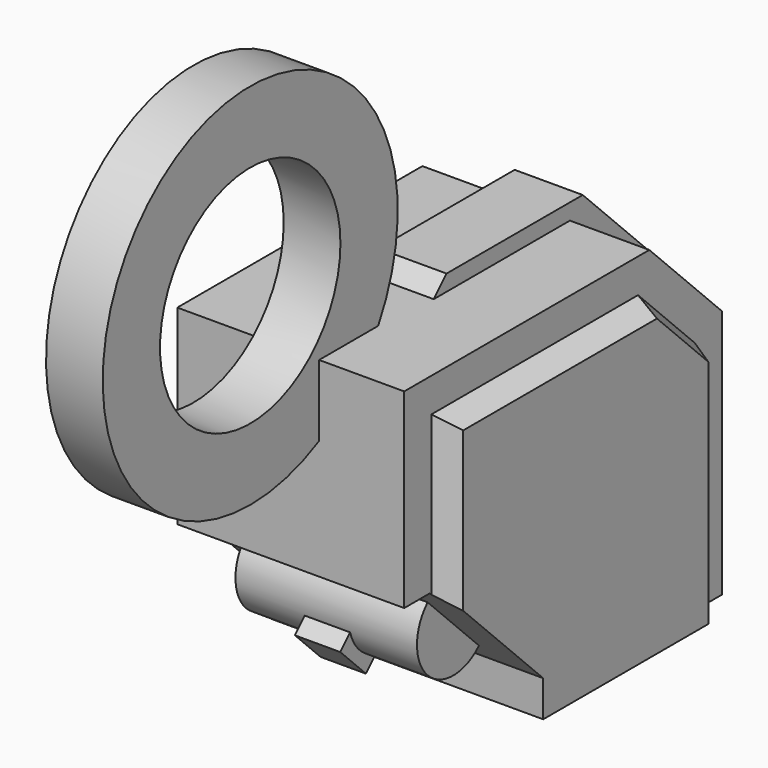
from build123d import *

# Parameters (mm, degrees)
F2_DEPTH       = 20
F3_DEPTH       = 22
F3_DEPTH_BACK  = 2
F1_W           = 29
F1_H           = 3
F7_DEPTH       = 22
F7_DEPTH_BACK  = 2
F5_W           = 6
F5_H           = 11.313708499
F4_W           = 6
F4_H           = 15
F6_W           = 6
F6_H           = 15
F8_DEPTH       = 2
F10_DEPTH      = 25
F12_DEPTH      = 5
F15_DEPTH      = 0.5
F16_R          = 16.2487088964
F16_R_2        = 9.9373882072
F17_DEPTH      = 2.5
F17_DEPTH_BACK = 2.5
F18_T4_DEPTH   = 31.116674808
F18_T9_DEPTH   = 19.1877426199
F18_T14_DEPTH  = 33.116674808
F18_T19_DEPTH  = 24.3595810189
F18_T24_DEPTH  = 24.3595810189
F18_T29_DEPTH  = 33.116674808
F18_T34_DEPTH  = 19.1877426199
F18_T39_DEPTH  = 31.116674808


# Not quite as in the source:
# - a fillet or chamfer that OpenCascade refuses, or shapes differently, is made with other operations: its cross-section is extruded or revolved along the edge and cut away or added
# - two fillets or chamfers of one size are made in one step


with BuildPart() as f2:
    # F1 (on Right) → F2 (new body)
    with BuildSketch(Plane.YZ):
        Polygon((-35, 30), (-35, 0), (-32, 0), (-32, 3), (-32, 27), (-9.2426406871, 27), (-3, 20.7573593129), (-3, 3), (-3, 0), (0, 0), (0, 22), (-8, 30), align=None)
    extrude(amount=F2_DEPTH)

    # F1 (on Right) → F3 (join, two sides)
    with BuildSketch(Plane.YZ) as f3_sk:
        Polygon((-32, 27), (-32, 3), (-3, 3), (-3, 20.7573593129), (-9.2426406871, 27), align=None)
    extrude(amount=F3_DEPTH)
    extrude(f3_sk.sketch, amount=-F3_DEPTH_BACK)

    # F1 (on Right) → F7 (join, two sides)
    with BuildSketch(Plane.YZ) as f7_sk:
        with Locations((-17.5, 1.5)):
            Rectangle(F1_W, F1_H)
    extrude(amount=F7_DEPTH)
    extrude(f7_sk.sketch, amount=-F7_DEPTH_BACK)

    # F5 (on face) + F4 (on face) + F6 (on face) → F8 (join)
    with BuildSketch(Plane(origin=(0, 11, 11), x_dir=(-1, 0, 0), z_dir=(0, 0.7071067812, 0.7071067812))):
        with Locations((-10, 21.2132034356)):
            Rectangle(F5_W, F5_H)
    with BuildSketch(Plane(origin=(0, 0, 0), x_dir=(-1, 0, 0), z_dir=(0, 1, 0))):
        with Locations((-10, 14.5)):
            Rectangle(F4_W, F4_H)
    with BuildSketch(Plane.XY.offset(30)):
        with Locations((10, -15.5)):
            Rectangle(F6_W, F6_H)
    extrude(amount=F8_DEPTH, dir=(0, 0.7071067812, 0.7071067812))

    # F9 (on face) → F10 (cut)
    with BuildSketch(Plane(origin=(-2, 0, 0), x_dir=(0, -1, 0), z_dir=(-1, 0, 0))):
        Polygon((22.18895033, -6.8113151938), (42.18895033, -6.8113151938), (42.18895033, 13.1886848062), (32.18895033, 13.1886848062), (32, 12.9997344762), (32, 0), (22.18895033, 0), align=None)
        Polygon((22.18895033, 3.1886848062), (22.18895033, 0), (32, 0), (32, 12.9997344762), align=None)
    extrude(amount=-F10_DEPTH, mode=Mode.SUBTRACT)

    # F11 (on face) → F12 (join)
    with BuildSketch(Plane(origin=(0, -9.5001327619, -9.5001327619), x_dir=(1, 0, 0), z_dir=(0, -0.7071067812, -0.7071067812))):
        Polygon((8, 26.8821576475), (8, 24.8821576475), (8, 22.8821576475), (12, 22.8821576475), (12, 24.8821576475), (12, 26.8821576475), align=None)
    extrude(amount=F12_DEPTH)

    # F11 (on face) → F13 (revolve)
    with BuildSketch(Plane(origin=(0, -9.5001327619, -9.5001327619), x_dir=(1, 0, 0), z_dir=(0, -0.7071067812, -0.7071067812))):
        Polygon((2, 28.8821576475), (2, 24.8821576475), (8, 24.8821576475), (8, 26.8821576475), (12, 26.8821576475), (12, 24.8821576475), (18, 24.8821576475), (18, 28.8821576475), align=None)
    revolve(axis=Axis((5, -27.094475165, 8.0942096412), (1, 0, 0)))

    # F14 (on face) → F15 (join)
    with BuildSketch(Plane(origin=(0, 1.4142135624, 0), x_dir=(-1, 0, 0), z_dir=(0, 1, 0))):
        with BuildLine():
            Line((-12, 21.4142135624), (-12, 10.4142135624))
            ThreePointArc((-12, 10.4142135624), (-11.7071067812, 9.7071067812), (-11, 9.4142135624))
            Line((-11, 9.4142135624), (-9, 9.4142135624))
            ThreePointArc((-9, 9.4142135624), (-8.2928932188, 9.7071067812), (-8, 10.4142135624))
            Line((-8, 10.4142135624), (-8, 21.4142135624))
            ThreePointArc((-8, 21.4142135624), (-8.2928932188, 22.1213203436), (-9, 22.4142135624))
            Line((-9, 22.4142135624), (-11, 22.4142135624))
            ThreePointArc((-11, 22.4142135624), (-11.7071067812, 22.1213203436), (-12, 21.4142135624))
        make_face()
    extrude(amount=F15_DEPTH)

    # F16 (on offset) → F17 (join, two sides)
    with BuildSketch(Plane.YZ.offset(10)) as f17_sk:
        with Locations((-42.5896607339, 38.0838625133)):
            Circle(F16_R)
        with Locations((-42.5896607339, 38.0838625133)):
            Circle(F16_R_2, mode=Mode.SUBTRACT)
    extrude(amount=F17_DEPTH)
    extrude(f17_sk.sketch, amount=-F17_DEPTH_BACK)

    # F18: chamfer of 2 x 1 on 8 edges, made by hand


with BuildPart() as f18_tool2:
    # F18_s3 → F18_t4 (new body)
    with BuildSketch(Plane.XY.offset(-5.1796577476)):
        Polygon((0, -3), (-2, -4), (-2, -3), align=None)
    extrude(amount=F18_T4_DEPTH)

    split(bisect_by=Plane.YZ, keep=Keep.BOTTOM)


with BuildPart() as f2_1:
    add(f2.part)

    # F18_t1: cut F18_tool2
    add(f18_tool2.part, mode=Mode.SUBTRACT)


with BuildPart() as f18_tool7:
    # F18_s8 → F18_t9 (new body)
    with BuildSketch(Plane(origin=(0, -8.2161085389, 8.2161085389), x_dir=(1, 0, 0), z_dir=(0, -0.7071067812, 0.7071067812))):
        Polygon((0, 12.5563491861), (-2, 11.5563491861), (-2, 12.5563491861), align=None)
    extrude(amount=F18_T9_DEPTH)

    split(bisect_by=Plane.YZ, keep=Keep.BOTTOM)


with BuildPart() as f2_2:
    add(f2_1.part)

    # F18_t6: cut F18_tool7
    add(f18_tool7.part, mode=Mode.SUBTRACT)


with BuildPart() as f18_tool12:
    # F18_s13 → F18_t14 (new body)
    with BuildSketch(Plane.XZ.offset(4.0629829395)):
        Polygon((0, 27), (-2, 26), (-2, 27), align=None)
    extrude(amount=F18_T14_DEPTH)

    split(bisect_by=Plane.YZ, keep=Keep.BOTTOM)


with BuildPart() as f2_3:
    add(f2_2.part)

    # F18_t11: cut F18_tool12
    add(f18_tool12.part, mode=Mode.SUBTRACT)


with BuildPart() as f18_tool17:
    # F18_s18 → F18_t19 (new body)
    with BuildSketch(Plane.XY.offset(32.1796577476)):
        Polygon((0, -32), (-2, -31), (-2, -32), align=None)
    extrude(amount=-F18_T19_DEPTH)

    split(bisect_by=Plane.YZ, keep=Keep.BOTTOM)


with BuildPart() as f2_4:
    add(f2_3.part)

    # F18_t16: cut F18_tool17
    add(f18_tool17.part, mode=Mode.SUBTRACT)


with BuildPart() as f18_tool22:
    # F18_s23 → F18_t24 (new body)
    with BuildSketch(Plane.XY.offset(7.8200767286)):
        Polygon((20, -32), (22, -31), (22, -32), align=None)
    extrude(amount=F18_T24_DEPTH)

    split(bisect_by=Plane.YZ.offset(20), keep=Keep.TOP)


with BuildPart() as f2_5:
    add(f2_4.part)

    # F18_t21: cut F18_tool22
    add(f18_tool22.part, mode=Mode.SUBTRACT)


with BuildPart() as f18_tool27:
    # F18_s28 → F18_t29 (new body)
    with BuildSketch(Plane.XZ.offset(4.0629829395)):
        Polygon((20, 27), (22, 26), (22, 27), align=None)
    extrude(amount=F18_T29_DEPTH)

    split(bisect_by=Plane.YZ.offset(20), keep=Keep.TOP)


with BuildPart() as f2_6:
    add(f2_5.part)

    # F18_t26: cut F18_tool27
    add(f18_tool27.part, mode=Mode.SUBTRACT)


with BuildPart() as f18_tool32:
    # F18_s33 → F18_t34 (new body)
    with BuildSketch(Plane(origin=(0, -8.2161085389, 8.2161085389), x_dir=(1, 0, 0), z_dir=(0, -0.7071067812, 0.7071067812))):
        Polygon((20, 12.5563491861), (22, 11.5563491861), (22, 12.5563491861), align=None)
    extrude(amount=F18_T34_DEPTH)

    split(bisect_by=Plane.YZ.offset(20), keep=Keep.TOP)


with BuildPart() as f2_7:
    add(f2_6.part)

    # F18_t31: cut F18_tool32
    add(f18_tool32.part, mode=Mode.SUBTRACT)


with BuildPart() as f18_tool37:
    # F18_s38 → F18_t39 (new body)
    with BuildSketch(Plane.XY.offset(25.9370170605)):
        Polygon((22, -4), (20, -3), (22, -3), align=None)
    extrude(amount=-F18_T39_DEPTH)

    split(bisect_by=Plane.YZ.offset(20), keep=Keep.TOP)


with BuildPart() as f2_8:
    add(f2_7.part)

    # F18_t36: cut F18_tool37
    add(f18_tool37.part, mode=Mode.SUBTRACT)


solid = f2_8.part
